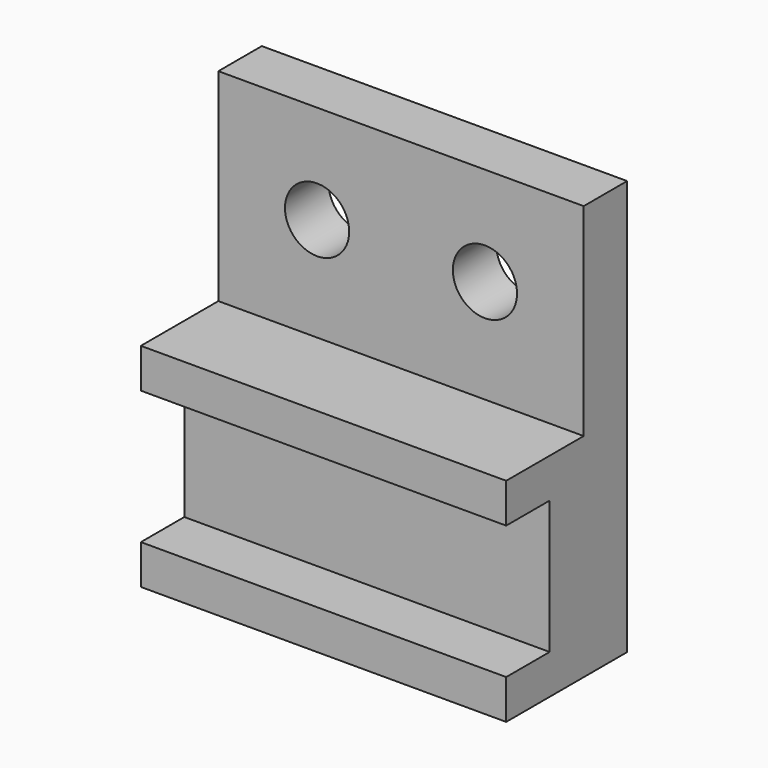
from build123d import *

# Parameters (mm, degrees)
F1_DEPTH = 117.475
F3_D     = 20.6375


# Not quite as in the source:
# - a length typed as a fraction of an inch, garbled in the dataset ("3 / 203.2 mm" for 3/8 in), is restored


with BuildPart() as f1:
    # F0 (on Right) → F1 (new body)
    with BuildSketch(Plane.YZ):
        Polygon((-51.1705551147, 49.2858837724), (-51.1705551147, 182.6358837724), (-68.6330551147, 182.6358837724), (-68.6330551147, 117.5483837724), (-68.6330551147, 49.2858837724), align=None)
        Polygon((-99.7797900677, 49.2858837724), (-68.6330551147, 49.2858837724), (-68.6330551147, 117.5483837724), (-99.7797900677, 117.5483837724), (-99.7797900677, 104.8483837724), (-82.3172900677, 104.8483837724), (-82.3172900677, 61.9858837724), (-99.7797900677, 61.9858837724), align=None)
    extrude(amount=F1_DEPTH)

    # F3 (through all)
    with Locations(Plane(origin=(0, 0, 0), x_dir=(1, 0, 0), z_dir=(0, 1, 0))):
        with Locations((31.75, -150.8858837724), (85.725, -150.8858837724)):
            Hole(F3_D / 2)


solid = f1.part
